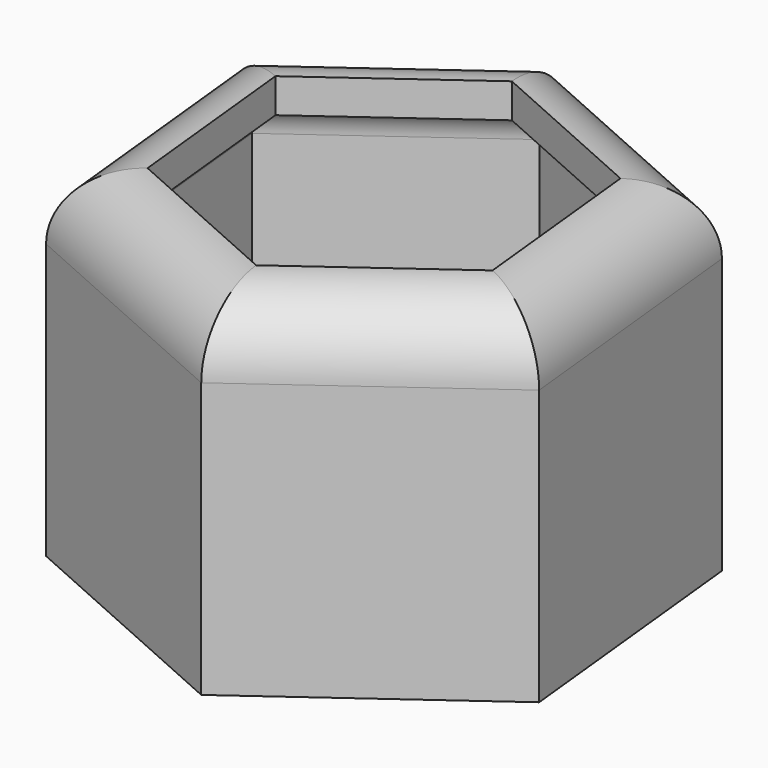
from build123d import *

# Parameters (mm, degrees)
F1_DEPTH = 25.4
F2_R     = 5.08
F3_T     = -2.54


# Not quite as in the source:
# - a shell that OpenCascade refuses in one call is made with other operations: the cavity is built on its own and cut out


with BuildPart() as f1:
    # F0 (on Top) → F1 (new body)
    with BuildSketch(Plane.XY):
        Polygon((-25.0890052673, 10.3711288533), (-9.2777067069, 21.8420710304), (-11.3061847575, 41.2705283392), (-29.1459613684, 49.2280434707), (-44.9572599288, 37.7571012935), (-42.9287818782, 18.3286439848), align=None)
    extrude(amount=F1_DEPTH)

    # F2
    f2_edges = [f1.edges().sort_by_distance(p)[0] for p in [
        (-37.051611, 43.492572, 25.4),
        (-20.226073, 45.249286, 25.4),
        (-10.291946, 31.5563, 25.4),
        (-17.183356, 16.1066, 25.4),
        (-34.008894, 14.349886, 25.4),
        (-43.943021, 28.042873, 25.4),
    ]]
    fillet(f2_edges, radius=F2_R)

    # F3: a shell. OpenCascade refuses it in one call, so the cavity is built on its own and cut out:
    # the body offset inwards by the wall thickness, plus a prism from it out through each open face.
    f3_core = offset(f1.part, amount=F3_T, mode=Mode.PRIVATE)
    f3_exits = [f3_core.faces().sort_by_distance(p)[0] for p in [
        (-27.117483, 29.799586, 22.86),
    ]]
    add(f3_core, mode=Mode.SUBTRACT)
    extrude(f3_exits, amount=-F3_T, mode=Mode.SUBTRACT)


solid = f1.part
